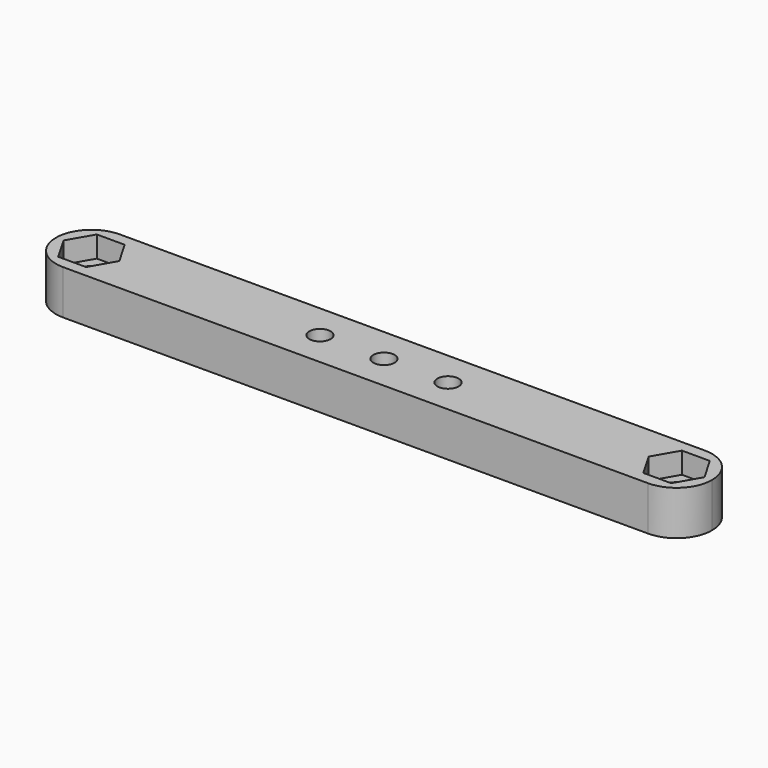
from build123d import *

# Parameters (mm, degrees)
F2_W      = 74
F2_H      = 8
F2_R      = 3
F5_DEPTH  = 5
F0_R      = 1.7
F6_DEPTH  = 12.5
F3_R      = 2.05
F7_DEPTH  = 2
F8_DEPTH  = 2
F10_DEPTH = 2.4
F11_R     = 3.99999
F4_R      = 1.2
F12_DEPTH = 5.001


# Not quite as in the source:
# - a fillet or chamfer is up to 0.001 mm smaller than in the source, because OpenCascade refuses the exact size


with BuildPart() as f5:
    # F2 (on face) → F5 (new body)
    with BuildSketch(Plane.XY):
        with Locations((0, 38)):
            Rectangle(F2_W, F2_H)
        with Locations((-33, 38)):
            Circle(F2_R, mode=Mode.SUBTRACT)
        Polygon((1.1402667816, 36.025), (0, 36.025), (-1.1402667816, 36.025), (-2.2805335633, 38), (-1.1402667816, 39.975), (0, 39.975), (1.1402667816, 39.975), (2.2805335633, 38), align=None, mode=Mode.SUBTRACT)
        with Locations((33, 38)):
            Circle(F2_R, mode=Mode.SUBTRACT)
        Polygon((-1.1402667816, 36.025), (0, 36.025), (1.1402667816, 36.025), (2.2805335633, 38), (1.1402667816, 39.975), (0, 39.975), (-1.1402667816, 39.975), (-2.2805335633, 38), align=None)
        with Locations((-33, 38)):
            Circle(F2_R)
        with Locations((33, 38)):
            Circle(F2_R)
    extrude(amount=F5_DEPTH)

    # F0 (on Top) → F6 (cut, symmetric)
    with BuildSketch(Plane.XY):
        with Locations((-33, 38)):
            Circle(F0_R)
        with Locations((33, 38)):
            Circle(F0_R)
        with Locations((-33, -38)):
            Circle(F0_R)
        with Locations((33, -38)):
            Circle(F0_R)
    extrude(amount=F6_DEPTH, both=True, mode=Mode.SUBTRACT)

    # F3 (on face) → F7 (cut)
    with BuildSketch(Plane.XY):
        with Locations((-7.225, 38)):
            Circle(F3_R)
        with Locations((7.225, 38)):
            Circle(F3_R)
    extrude(amount=F7_DEPTH, mode=Mode.SUBTRACT)

    # F2 (on face) → F8 (cut)
    with BuildSketch(Plane.XY):
        Polygon((-1.1402667816, 36.025), (0, 36.025), (1.1402667816, 36.025), (2.2805335633, 38), (1.1402667816, 39.975), (0, 39.975), (-1.1402667816, 39.975), (-2.2805335633, 38), align=None)
    extrude(amount=F8_DEPTH, mode=Mode.SUBTRACT)

    # F9 (on face) → F10 (cut)
    with BuildSketch(Plane.XY.offset(5)):
        Polygon((-34.5732794835, 35.275), (-33, 35.275), (-31.4267205165, 35.275), (-29.8534410329, 38), (-31.4267205165, 40.725), (-33, 40.725), (-34.5732794835, 40.725), (-36.1465589671, 38), align=None)
        Polygon((29.8534410329, 38), (31.4267205165, 35.275), (33, 35.275), (34.5732794835, 35.275), (36.1465589671, 38), (34.5732794835, 40.725), (33, 40.725), (31.4267205165, 40.725), align=None)
    extrude(amount=-F10_DEPTH, mode=Mode.SUBTRACT)

    # F11 (radius 4 in the source; OpenCascade refuses exactly that, so slightly less here)
    f11_edges = [f5.edges().sort_by_distance(p)[0] for p in [
        (-37, 42, 2.5),
        (-37, 34, 2.5),
        (37, 42, 2.5),
        (37, 34, 2.5),
    ]]
    fillet(f11_edges, radius=F11_R)

    # F4 (on face) → F12 (cut, through all)
    with BuildSketch(Plane.XY):
        with Locations((-7.225, 38)):
            Circle(F4_R)
        with Locations((0, 38)):
            Circle(F4_R)
        with Locations((7.225, 38)):
            Circle(F4_R)
    extrude(amount=F12_DEPTH, mode=Mode.SUBTRACT)


solid = f5.part
